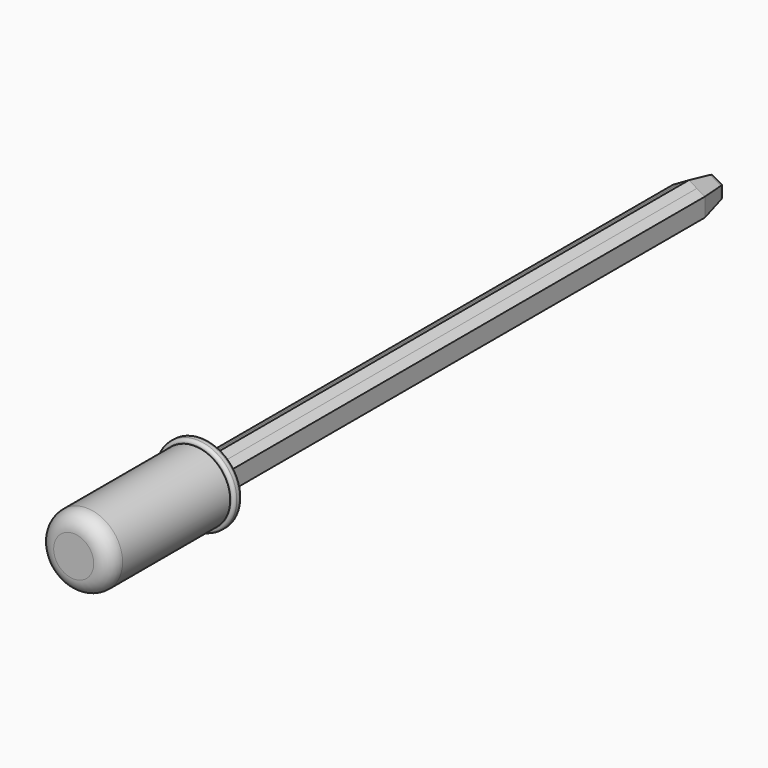
from build123d import *

# Parameters (mm, degrees)
F1_DEPTH    = 200
F2_R        = 11.25
F3_DEPTH    = 50
F4_R        = 12.5
F5_DEPTH    = 3
F6_R        = 1
F7_R        = 5
F8_T1_DEPTH = 57.7361444178
F8_T3_DEPTH = 57.7361444178
F8_T5_DEPTH = 57.7361444178
F8_T7_DEPTH = 57.7361444178
F8_T9_DEPTH = 57.7361444178
F9_T1_DEPTH = 11.6621406423
F9_T3_DEPTH = 11.6621406423
F9_T5_DEPTH = 11.6621406423
F9_T7_DEPTH = 11.6621406423


# Not quite as in the source:
# - a fillet or chamfer that OpenCascade refuses, or shapes differently, is made with other operations: its cross-section is extruded or revolved along the edge and cut away or added


with BuildPart() as f1:
    # F0 (on Front) → F1 (new body)
    with BuildSketch(Plane.XZ):
        with BuildLine():
            ThreePointArc((2.5000000636, -4.3301269822), (4.3301270373, -2.4999999682), (5, 0))
            ThreePointArc((5, 0), (4.3301270373, 2.4999999682), (2.5000000636, 4.3301269822))
            ThreePointArc((2.5000000636, 4.3301269822), (1.215e-07, 5), (-2.4999998532, 4.3301271037))
            ThreePointArc((-2.4999998532, 4.3301271037), (-4.3301269765, 2.5000000734), (-5, 0))
            ThreePointArc((-5, 0), (-4.3301270351, -2.4999999721), (-2.5000000559, -4.3301269867))
            ThreePointArc((-2.5000000559, -4.3301269867), (4.5e-09, -5), (2.5000000636, -4.3301269822))
        make_face()
        with BuildLine():
            Line((5, -2.8867513459), (5, 0))
            ThreePointArc((5, 0), (4.3301270373, -2.4999999682), (2.5000000636, -4.3301269822))
            Line((2.5000000636, -4.3301269822), (5, -2.8867513459))
        make_face()
        with BuildLine():
            ThreePointArc((2.5000000636, 4.3301269822), (4.3301270373, 2.4999999682), (5, 0))
            Line((5, 0), (5, 2.8867513459))
            Line((5, 2.8867513459), (2.5000000636, 4.3301269822))
        make_face()
        with BuildLine():
            ThreePointArc((-2.4999998532, 4.3301271037), (1.215e-07, 5), (2.5000000636, 4.3301269822))
            Line((2.5000000636, 4.3301269822), (0, 5.7735026919))
            Line((0, 5.7735026919), (-2.4999998532, 4.3301271037))
        make_face()
        with BuildLine():
            Line((0, -5.7735026919), (2.5000000636, -4.3301269822))
            ThreePointArc((2.5000000636, -4.3301269822), (4.5e-09, -5), (-2.5000000559, -4.3301269867))
            Line((-2.5000000559, -4.3301269867), (0, -5.7735026919))
        make_face()
        with BuildLine():
            ThreePointArc((-5, 0), (-4.3301269765, 2.5000000734), (-2.4999998532, 4.3301271037))
            Line((-2.4999998532, 4.3301271037), (-5, 2.8867513459))
            Line((-5, 2.8867513459), (-5, 0))
        make_face()
        with BuildLine():
            Line((-5, -2.8867513459), (-2.5000000559, -4.3301269867))
            ThreePointArc((-2.5000000559, -4.3301269867), (-4.3301270351, -2.4999999721), (-5, 0))
            Line((-5, 0), (-5, -2.8867513459))
        make_face()
    extrude(amount=F1_DEPTH)

    # F2 (on face) → F3 (join)
    with BuildSketch(Plane.XZ.offset(200)):
        Circle(F2_R)
    extrude(amount=F3_DEPTH)

    # F4 (on face) → F5 (join)
    with BuildSketch(Plane(origin=(0, -200, 0), x_dir=(-1, 0, 0), z_dir=(0, 1, 0))):
        Circle(F4_R)
    extrude(amount=-F5_DEPTH)

    # F6
    f6_edges = [f1.edges().sort_by_distance(p)[0] for p in [
        (12.5, -203, 0),
        (12.5, -200, 0),
    ]]
    fillet(f6_edges, radius=F6_R)

    # F7
    f7_edges = [f1.edges().sort_by_distance(p)[0] for p in [
        (-11.25, -250, 0),
    ]]
    fillet(f7_edges, radius=F7_R)

    # F8: chamfer of 2 x 10 on 6 edges, made by hand

    # F8_s2 → F8_t1 (cut)
    with BuildSketch(Plane.XY.offset(-28.8680722089)):
        Polygon((5, -10), (3, 0), (5, 0), align=None)
        Polygon((-5, -10), (-3, 0), (-5, 0), align=None)
    extrude(amount=F8_T1_DEPTH, mode=Mode.SUBTRACT)

    # F8_s4 → F8_t3 (cut)
    with BuildSketch(Plane(origin=(25.0004838912, 0, -14.4340361045), x_dir=(0, 1, 0), z_dir=(-0.8660254038, 0, 0.5))):
        Polygon((-10, -5), (0, -3), (0, -5), align=None)
    extrude(amount=F8_T3_DEPTH, mode=Mode.SUBTRACT)

    # F8_s6 → F8_t5 (cut)
    with BuildSketch(Plane(origin=(25.0004838912, 0, 14.4340361045), x_dir=(0, 1, 0), z_dir=(-0.8660254038, 0, -0.5))):
        Polygon((-10, -5), (0, -3), (0, -5), align=None)
    extrude(amount=F8_T5_DEPTH, mode=Mode.SUBTRACT)

    # F8_s8 → F8_t7 (cut)
    with BuildSketch(Plane(origin=(-25.0004838912, 0, 14.4340361045), x_dir=(0, 1, 0), z_dir=(0.8660254038, 0, -0.5))):
        Polygon((-10, -5), (0, -3), (0, -5), align=None)
    extrude(amount=F8_T7_DEPTH, mode=Mode.SUBTRACT)

    # F8_s10 → F8_t9 (cut)
    with BuildSketch(Plane(origin=(-25.0004838912, 0, -14.4340361045), x_dir=(0, 1, 0), z_dir=(0.8660254038, 0, 0.5))):
        Polygon((-10, -5), (0, -3), (0, -5), align=None)
    extrude(amount=F8_T9_DEPTH, mode=Mode.SUBTRACT)

    # F9: fillet of radius 2 on 5 edges, made by hand

    # F9_s2 → F9_t1 (cut)
    with BuildSketch(Plane.XY.offset(-5.8310703212)):
        with BuildLine():
            ThreePointArc((3.3215535459, -1.6077677297), (2.6283700058, -0.4533157173), (1.3603921946, 0))
            Line((1.3603921946, 0), (3, 0))
            Line((3, 0), (3.3215535459, -1.6077677297))
        make_face()
        with BuildLine():
            ThreePointArc((-3.3215535459, -1.6077677297), (-2.6283700058, -0.4533157173), (-1.3603921946, 0))
            Line((-1.3603921946, 0), (-3, 0))
            Line((-3, 0), (-3.3215535459, -1.6077677297))
        make_face()
    extrude(amount=F9_T1_DEPTH, mode=Mode.SUBTRACT)

    # F9_s4 → F9_t3 (cut)
    with BuildSketch(Plane(origin=(5.0498550294, 0, 2.9155351606), x_dir=(0, 1, 0), z_dir=(-0.8660254038, 0, -0.5))):
        with BuildLine():
            ThreePointArc((-1.6077677297, -3.3215535459), (-0.4533157173, -2.6283700058), (0, -1.3603921946))
            Line((0, -1.3603921946), (0, -3))
            Line((0, -3), (-1.6077677297, -3.3215535459))
        make_face()
    extrude(amount=F9_T3_DEPTH, mode=Mode.SUBTRACT)

    # F9_s6 → F9_t5 (cut)
    with BuildSketch(Plane(origin=(-5.0498550294, 0, 2.9155351606), x_dir=(0, 1, 0), z_dir=(0.8660254038, 0, -0.5))):
        with BuildLine():
            ThreePointArc((-1.6077677297, -3.3215535459), (-0.4533157173, -2.6283700058), (0, -1.3603921946))
            Line((0, -1.3603921946), (0, -3))
            Line((0, -3), (-1.6077677297, -3.3215535459))
        make_face()
    extrude(amount=F9_T5_DEPTH, mode=Mode.SUBTRACT)

    # F9_s8 → F9_t7 (cut)
    with BuildSketch(Plane(origin=(5.0498550294, 0, -2.9155351606), x_dir=(0, 1, 0), z_dir=(-0.8660254038, 0, 0.5))):
        with BuildLine():
            ThreePointArc((-1.6077677297, -3.3215535459), (-0.4533157173, -2.6283700058), (0, -1.3603921946))
            Line((0, -1.3603921946), (0, -3))
            Line((0, -3), (-1.6077677297, -3.3215535459))
        make_face()
    extrude(amount=F9_T7_DEPTH, mode=Mode.SUBTRACT)


solid = f1.part
